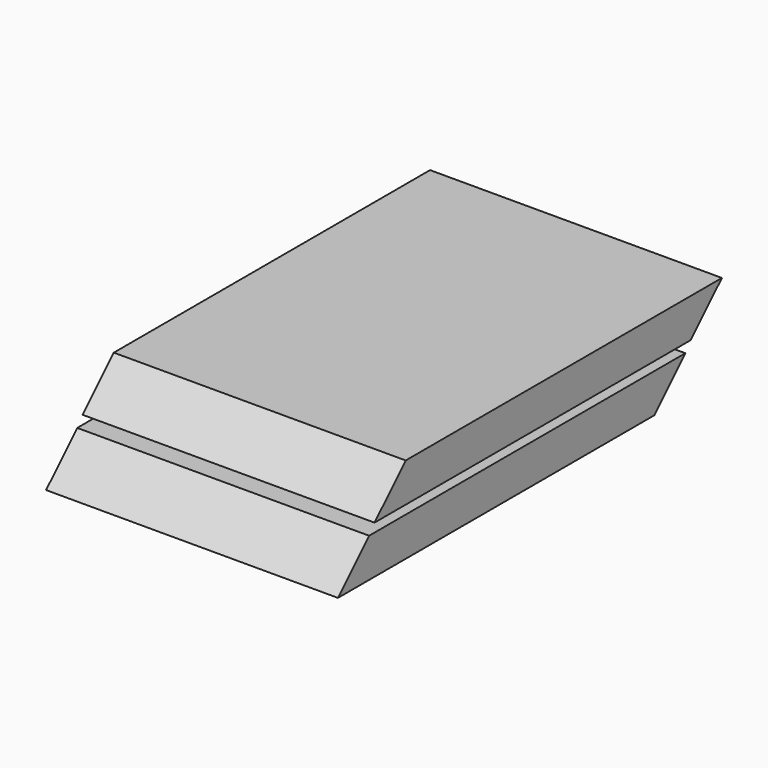
from build123d import *

# Parameters (mm, degrees)
F0_W        = 152.4
F0_H        = 236.8748463745
F1_DEPTH    = 20.32
F2_T1_DEPTH = 283.0414957887
F3_T1_DEPTH = 283.0414957887


# Not quite as in the source:
# - a fillet or chamfer that OpenCascade refuses, or shapes differently, is made with other operations: its cross-section is extruded or revolved along the edge and cut away or added
# - the program builds the solid bodies; features that only make, move or delete a surface that nothing else refers to are left out


with BuildPart() as f1:
    # F0 (on Top) → F1 (new body)
    with BuildSketch(Plane.XY):
        with Locations((-0.1412853599, 42.7363403141)):
            Rectangle(F0_W, F0_H)
    extrude(amount=F1_DEPTH)

    # F2: chamfer of 25.4 on 1 edges, made by hand

    # F2_s2 → F2_t1 (cut)
    with BuildSketch(Plane.YZ.offset(-141.6620332542)):
        Polygon((-75.7010828731, -5.08), (-50.3010828731, 20.32), (-75.7010828731, 20.32), align=None)
    extrude(amount=F2_T1_DEPTH, mode=Mode.SUBTRACT)

    # F3: chamfer of 25.4 on 1 edges, made by hand

    # F3_s2 → F3_t1 (cut)
    with BuildSketch(Plane.YZ.offset(-141.6620332542)):
        Polygon((161.1737635014, 25.4), (135.7737635014, 0), (161.1737635014, 0), align=None)
    extrude(amount=F3_T1_DEPTH, mode=Mode.SUBTRACT)


with BuildPart() as f4_1:
    # F4: copy of F1
    add(f1.part.moved(Location((0, 23.876, 24.892))))


solid = Compound([f1.part, f4_1.part])
